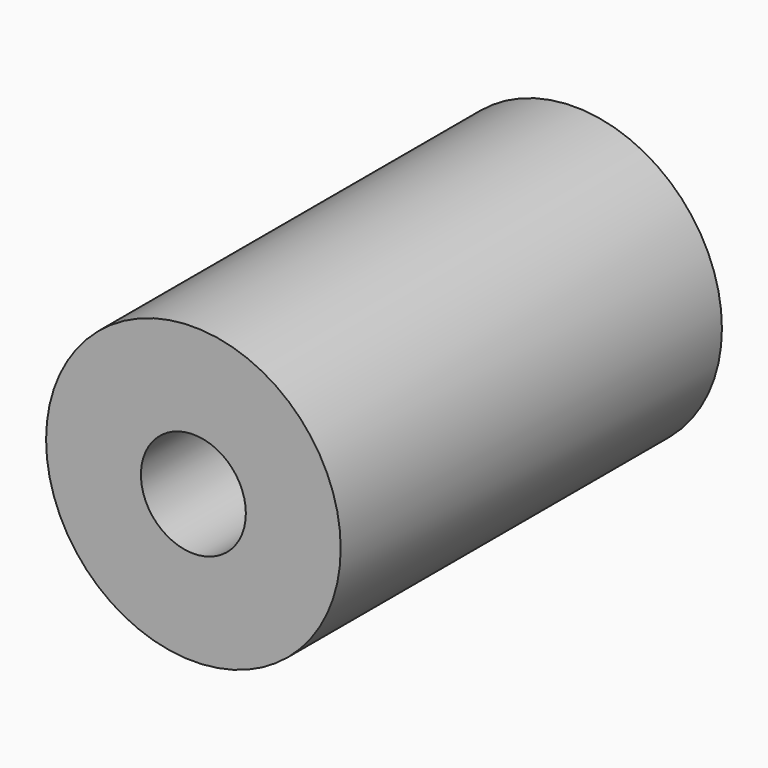
from build123d import *

# Parameters (mm, degrees)
F0_R     = 38.9485582709
F0_R_2   = 13.8718945382
F1_DEPTH = 63


# Not quite as in the source:
# - a feature names something its author has since deleted; it is built from what else it names


with BuildPart() as f1:
    # F0 (on Front) → F1 (new body, symmetric)
    with BuildSketch(Plane.XZ):
        with Locations((0, -54.3005429208)):
            Circle(F0_R)
        with Locations((0, -54.3005429208)):
            Circle(F0_R_2, mode=Mode.SUBTRACT)
    extrude(amount=F1_DEPTH, both=True)


solid = f1.part
